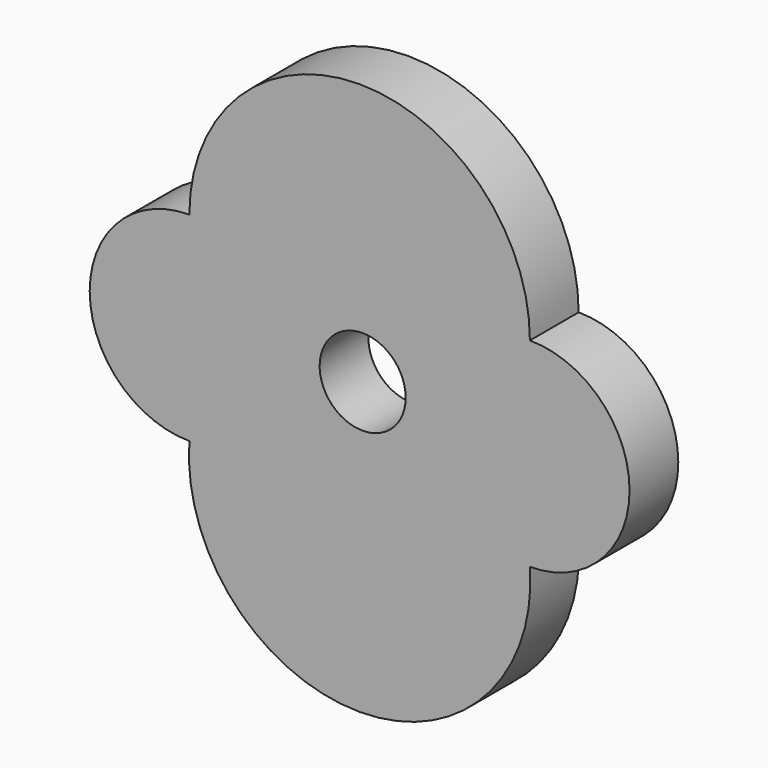
from build123d import *

# Parameters (mm, degrees)
F1_DEPTH = 25.4


with BuildPart() as f1:
    # F0 (on Front) → F1 (new body)
    with BuildSketch(Plane.XZ):
        with BuildLine():
            ThreePointArc((69.7280094028, 37.8677658737), (-1.2611225247, 108.8568978012), (-72.2502544522, 37.8677658737))
            Line((-72.2502544522, 37.8677658737), (-51.3892844319, 37.8677658737))
            Line((-51.3892844319, 37.8677658737), (0, 37.8677658737))
            Line((0, 37.8677658737), (69.7280094028, 37.8677658737))
        make_face()
        Polygon((-51.3892844319, 37.8677658737), (-72.2502544522, 37.8677658737), (-72.2502544522, -45.2175028622), (69.7280094028, -45.2175028622), (69.7280094028, -29.6100229025), (-51.3892844319, -29.6100229025), align=None)
        with BuildLine():
            Line((-72.2502544522, -45.2175028622), (-72.2502544522, 37.8677658737))
            ThreePointArc((-72.2502544522, 37.8677658737), (-113.7928888202, -3.6748684943), (-72.2502544522, -45.2175028622))
        make_face()
        with BuildLine():
            Line((0, 37.8677658737), (-51.3892844319, 37.8677658737))
            Line((-51.3892844319, 37.8677658737), (-51.3892844319, -29.6100229025))
            Line((-51.3892844319, -29.6100229025), (69.7280094028, -29.6100229025))
            Line((69.7280094028, -29.6100229025), (69.7280094028, 0))
            Line((69.7280094028, 0), (17.9303269799, 0))
            ThreePointArc((17.9303269799, 0), (-12.6786557964, -12.6786557964), (0, 17.9303269799))
            Line((0, 17.9303269799), (0, 37.8677658737))
        make_face()
        with BuildLine():
            Line((69.7280094028, -45.2175028622), (-72.2502544522, -45.2175028622))
            ThreePointArc((-72.2502544522, -45.2175028622), (-1.2611225247, -121.5592398304), (69.7280094028, -45.2175028622))
        make_face()
        with BuildLine():
            Line((69.7280094028, 0), (69.7280094028, 37.8677658737))
            Line((69.7280094028, 37.8677658737), (0, 37.8677658737))
            Line((0, 37.8677658737), (0, 17.9303269799))
            ThreePointArc((0, 17.9303269799), (12.6786557964, 12.6786557964), (17.9303269799, 0))
            Line((17.9303269799, 0), (69.7280094028, 0))
        make_face()
        with BuildLine():
            ThreePointArc((69.7280094028, -45.2175028622), (111.2706437707, -3.6748684943), (69.7280094028, 37.8677658737))
            Line((69.7280094028, 37.8677658737), (69.7280094028, 0))
            Line((69.7280094028, 0), (69.7280094028, -29.6100229025))
            Line((69.7280094028, -29.6100229025), (69.7280094028, -45.2175028622))
        make_face()
    extrude(amount=F1_DEPTH)


solid = f1.part
